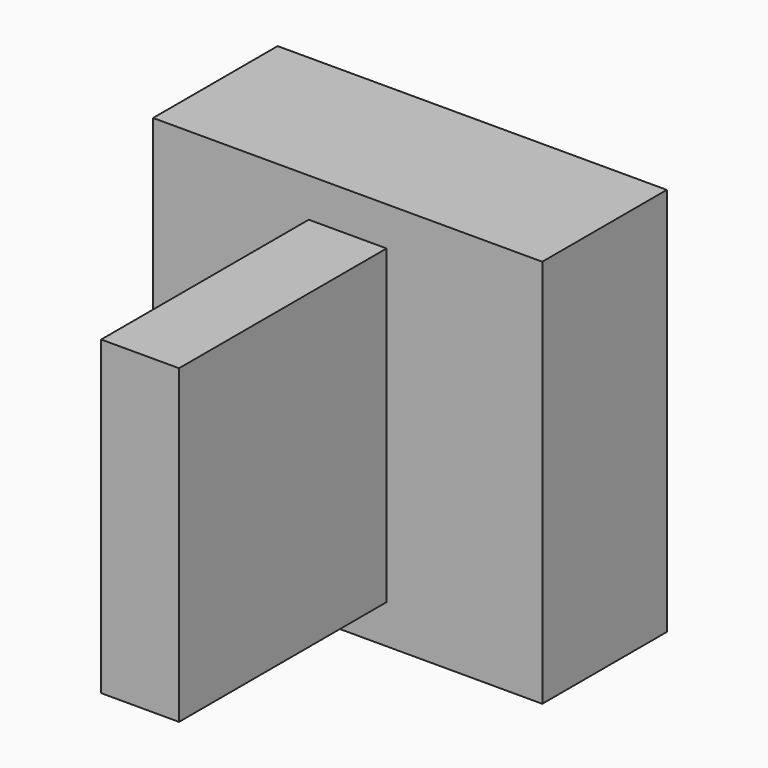
from build123d import *

# Parameters (mm, degrees)
F0_W     = 19.05
F0_H     = 19.05
F1_DEPTH = 7.62
F2_W     = 3.81
F2_H     = 15.24
F3_DEPTH = 2.54
F4_R     = 2.54
F5_DEPTH = 5.08
F6_DEPTH = 15.24


# Not quite as in the source:
# - a feature names something its author has since deleted; it is built from what else it names


with BuildPart() as f1:
    # F0 (on Front) → F1 (new body)
    with BuildSketch(Plane.XZ):
        with Locations((1.905, 9.525)):
            Rectangle(F0_W, F0_H)
    extrude(amount=F1_DEPTH)

    # F2 (on face) → F3 (cut)
    with BuildSketch(Plane.XZ.offset(7.62)):
        with Locations((1.905, 9.525)):
            Rectangle(F2_W, F2_H)
    extrude(amount=-F3_DEPTH, mode=Mode.SUBTRACT)

    # F4 (on face) → F5 (join)
    with BuildSketch(Plane(origin=(0, 0, 0), x_dir=(-1, 0, 0), z_dir=(0, 1, 0))):
        with Locations((-1.905, 9.525)):
            Circle(F4_R)
    extrude(amount=F5_DEPTH)


with BuildPart() as f6:
    # F6 (new): a face of the model
    f6_faces = [f1.part.faces().sort_by_distance(p)[0] for p in [
        (1.905, -5.08, 9.525),
    ]]
    extrude(f6_faces, amount=F6_DEPTH)


solid = Compound([f1.part, f6.part])
